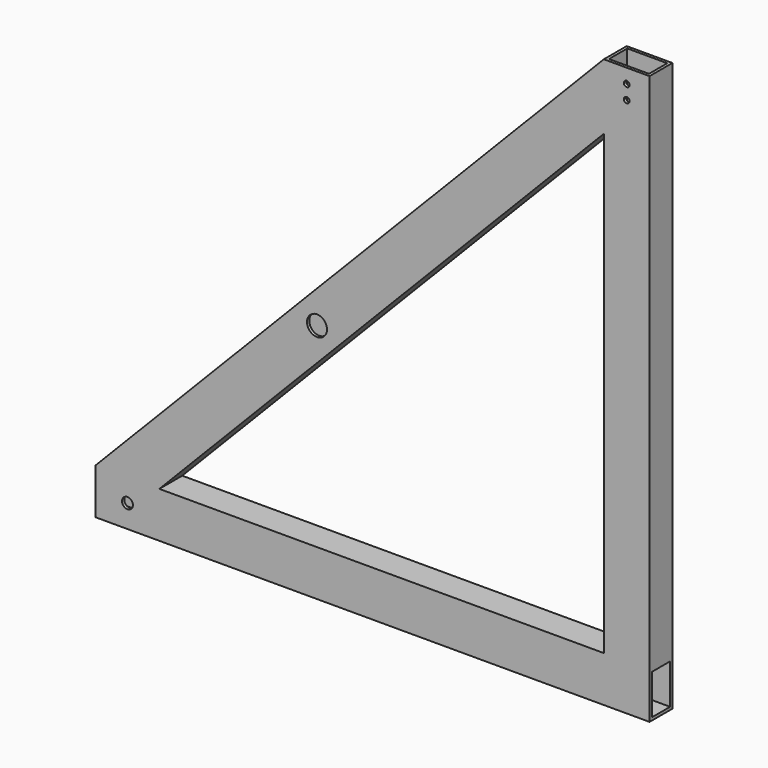
from build123d import *

# Parameters (mm, degrees)
F0_W         = 50
F0_H         = 80
F0_W_2       = 40
F0_H_2       = 70
F1_DEPTH     = 969
F2_W         = 80
F2_H         = 50
F2_W_2       = 70
F2_H_2       = 40
F3_DEPTH     = 914.4
F5_DEPTH     = 50
F6_R         = 17.5
F6_R_2       = 9.5
F7_DEPTH     = 50.001
F8_T         = 5
F8_T3_DEPTH  = 60
F8_T5_DEPTH  = 979
F8_T7_DEPTH  = 924.4
F8_T9_DEPTH  = 80
F8_T11_DEPTH = 50
F6_R_3       = 5
F9_DEPTH     = 5


# Not quite as in the source:
# - a shell that OpenCascade refuses in one call is made with other operations: the cavity is built on its own and cut out
# - a feature names something its author has since deleted; it is built from what else it names


with BuildPart() as f1:
    # F0 (on Right) → F1 (new body)
    with BuildSketch(Plane.YZ):
        with Locations((-25, 40)):
            Rectangle(F0_W, F0_H)
        with Locations((-25, 40)):
            Rectangle(F0_W_2, F0_H_2, mode=Mode.SUBTRACT)
    extrude(amount=-F1_DEPTH)

    # F2 (on face) → F3 (join)
    with BuildSketch(Plane.XY.offset(80)):
        with Locations((-40, -25)):
            Rectangle(F2_W, F2_H)
        with Locations((-40, -25)):
            Rectangle(F2_W_2, F2_H_2, mode=Mode.SUBTRACT)
    extrude(amount=F3_DEPTH)

    # F4 (on face) → F5 (join)
    with BuildSketch(Plane.XZ.offset(50)):
        Polygon((-80, 994.4), (-969, 80), (-857.4231981277, 80), (-80, 879.6352895028), align=None)
    extrude(amount=-F5_DEPTH)

    # F6 (on face) → F7 (cut, through all)
    with BuildSketch(Plane.XZ.offset(50)):
        with Locations((-581.6838212861, 421)):
            Circle(F6_R)
        with Locations((-913.2115990639, 40)):
            Circle(F6_R_2)
    extrude(amount=-F7_DEPTH, mode=Mode.SUBTRACT)

    # F8: shell of thickness 5, made by hand


with BuildPart() as f8_core1:
    # F8_t2: copy of F1
    add(f1.part)

    # the walls: a layer under each face that stays
    f8_faces = [f8_core1.faces().sort_by_distance(p)[0] for p in [
        (-484.5, -25, 0),
        (-484.5, -50, 497.2),
        (-484.5, 0, 497.2),
        (0, -25, 497.2),
        (-969, -46.4285714286, 5.7142857143),
        (-524.5, -25, 537.2),
        (-74.2857142857, -46.4285714286, 994.4),
        (-922.7115990639, -47.5, 40),
        (-468.7115990639, -25, 80),
        (-80, -25, 479.8176447514),
        (-468.7115990639, -25, 479.8176447514),
        (-922.7115990639, -2.5, 40),
        (-484.5, -25, 75),
        (-484.5, -5, 40),
        (-484.5, -25, 5),
        (-484.5, -45, 40),
        (-40, -5, 537.2),
        (-5, -25, 537.2),
        (-40, -45, 537.2),
        (-75, -25, 537.2),
        (-40, -25, 80),
    ]]
    thicken(f8_faces, amount=-F8_T, mode=Mode.SUBTRACT)

    # F8_s4 → F8_t3 (cut)
    with BuildSketch(Plane.XZ.offset(-5)):
        Polygon((-80.05, 80.05), (-80, 75), (-75, 75), (-75, 80), align=None)
        Polygon((-857.3873483818, 80.0151460803), (-857.4231981277, 75), (-869.2578593558, 75), (-861.0081727218, 83.4853919665), align=None)
        Polygon((-80.0141502541, 879.6004355831), (-75, 879.6352895028), (-75, 891.9509410517), (-83.5849745941, 883.1206814692), align=None)
    extrude(amount=F8_T3_DEPTH, mode=Mode.SUBTRACT)

    # F8_s6 → F8_t5 (cut)
    with BuildSketch(Plane.YZ.offset(-974)):
        Polygon((-44.95, 74.95), (-45, 80), (-50, 80), (-50, 75), align=None)
        Polygon((-5.05, 74.95), (-5, 80), (0, 80), (0, 75), align=None)
        Polygon((-5.05, 5.05), (0, 5), (0, 0), (-5, 0), align=None)
        Polygon((-44.95, 5.05), (-45, 0), (-50, 0), (-50, 5), align=None)
    extrude(amount=F8_T5_DEPTH, mode=Mode.SUBTRACT)

    # F8_s8 → F8_t7 (cut)
    with BuildSketch(Plane.XY.offset(75)):
        Polygon((-74.95, -5.05), (-75, 0), (-80, 0), (-80, -5), align=None)
        Polygon((-5.05, -5.05), (-5, 0), (0, 0), (0, -5), align=None)
        Polygon((-5.05, -44.95), (0, -45), (0, -50), (-5, -50), align=None)
        Polygon((-74.95, -44.95), (-75, -50), (-80, -50), (-80, -45), align=None)
    extrude(amount=F8_T7_DEPTH, mode=Mode.SUBTRACT)

    # F8_s10 → F8_t9 (cut)
    with BuildSketch(Plane.YZ.offset(-80)):
        Polygon((-5.05, 80.05), (0, 80), (0, 75), (-5, 75), align=None)
        Polygon((-44.95, 80.05), (-50, 80), (-50, 75), (-45, 75), align=None)
    extrude(amount=F8_T9_DEPTH, mode=Mode.SUBTRACT)

    # F8_s12 → F8_t11 (cut)
    with BuildSketch(Plane.XZ):
        Polygon((-5.05, 80.05), (0, 80), (0, 75), (-5, 75), align=None)
        Polygon((-74.95, 80.05), (-80, 80), (-80, 75), (-75, 75), align=None)
    extrude(amount=F8_T11_DEPTH, mode=Mode.SUBTRACT)


with BuildPart() as f1_1:
    add(f1.part)

    # what is left inside the walls is the cavity
    f8_cavity = [f8_core1.part.solids().sort_by_distance(p)[0] for p in [
        (-635.349987, -5.05, 363.508502),
    ]]
    add(f8_cavity, mode=Mode.SUBTRACT)

    # F6 (on face) → F9 (cut, through all)
    with BuildSketch(Plane.XZ.offset(50)):
        with Locations((-40, 969.4)):
            Circle(F6_R_3)
        with Locations((-40, 944.4)):
            Circle(F6_R_3)
    extrude(amount=-F9_DEPTH, mode=Mode.SUBTRACT)


solid = f1_1.part
